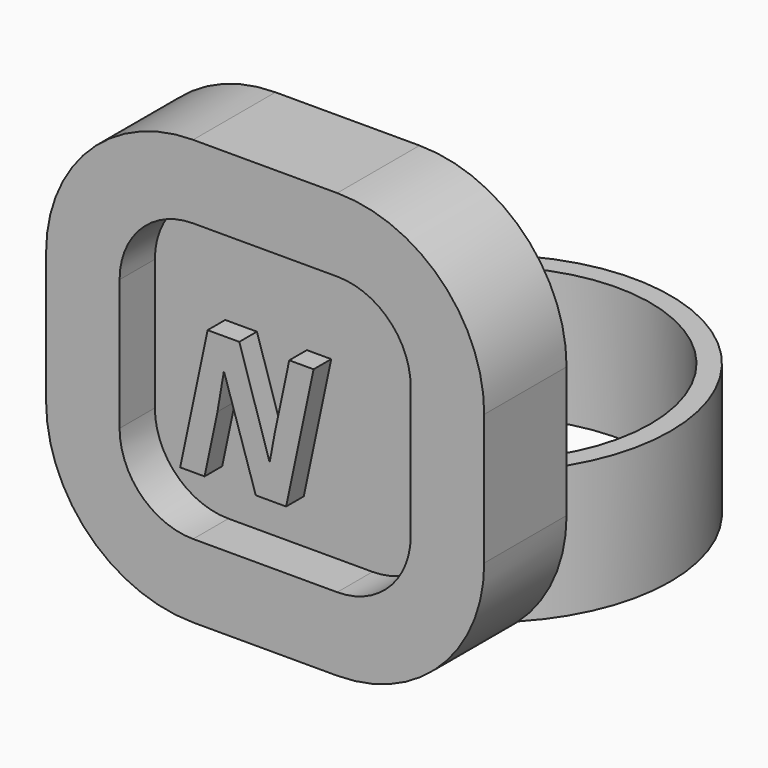
from build123d import *

# Parameters (mm, degrees)
F1_DEPTH     = 7
F2_DEPTH     = 4
F3_TEXT_SIZE = 12.3611111111
F4_DEPTH     = 1.5
F5_R         = 12.5
F5_R_2       = 11.15
F6_DEPTH     = 9


# Not quite as in the source:
# - a feature of the source that left no trace in its solid (it failed there, or was rolled back) is left out
# - Text() gives the source's letters only with a copy of the font that has no kerning and outlines rounded to 1/6400 em; it was checked with that copy


with BuildPart() as f1:
    # F0 (on Front) → F1 (new body)
    with BuildSketch(Plane.XZ):
        with BuildLine():
            Line((-90.7631201082, 7.9620657489), (-100.5631201082, 7.9620657489))
            ThreePointArc((-100.5631201082, 7.9620657489), (-107.6341876851, 5.0331336581), (-110.5631197759, -2.0379339188))
            Line((-110.5631197759, -2.0379339188), (-110.5631197759, -10.9379339188))
            ThreePointArc((-110.5631197759, -10.9379339188), (-107.6341876851, -18.0090014957), (-100.5631201082, -20.9379335865))
            Line((-100.5631201082, -20.9379335865), (-90.7631201082, -20.9379335865))
            ThreePointArc((-90.7631201082, -20.9379335865), (-83.6920525313, -18.0090014957), (-80.7631204405, -10.9379339188))
            Line((-80.7631204405, -10.9379339188), (-80.7631204405, -2.0379339188))
            ThreePointArc((-80.7631204405, -2.0379339188), (-83.6920525313, 5.0331336581), (-90.7631201082, 7.9620657489))
        make_face()
        with BuildLine():
            Line((-90.7631201082, -15.9379339188), (-100.5631201082, -15.9379339188))
            ThreePointArc((-100.5631201082, -15.9379339188), (-104.0986540141, -14.4734678248), (-105.5631201082, -10.9379339188))
            Line((-105.5631201082, -10.9379339188), (-105.5631201082, -2.0379339188))
            ThreePointArc((-105.5631201082, -2.0379339188), (-104.0986540141, 1.4975999871), (-100.5631201082, 2.9620660812))
            Line((-100.5631201082, 2.9620660812), (-90.7631201082, 2.9620660812))
            ThreePointArc((-90.7631201082, 2.9620660812), (-87.2275862022, 1.4975999871), (-85.7631201082, -2.0379339188))
            Line((-85.7631201082, -2.0379339188), (-85.7631201082, -10.9379339188))
            ThreePointArc((-85.7631201082, -10.9379339188), (-87.2275862022, -14.4734678248), (-90.7631201082, -15.9379339188))
        make_face(mode=Mode.SUBTRACT)
    extrude(amount=F1_DEPTH)

    # F0 (on Front) → F2 (join)
    with BuildSketch(Plane.XZ):
        with BuildLine():
            ThreePointArc((-105.5631201082, -10.9379339188), (-104.0986540141, -14.4734678248), (-100.5631201082, -15.9379339188))
            Line((-100.5631201082, -15.9379339188), (-90.7631201082, -15.9379339188))
            ThreePointArc((-90.7631201082, -15.9379339188), (-87.2275862022, -14.4734678248), (-85.7631201082, -10.9379339188))
            Line((-85.7631201082, -10.9379339188), (-85.7631201082, -2.0379339188))
            ThreePointArc((-85.7631201082, -2.0379339188), (-87.2275862022, 1.4975999871), (-90.7631201082, 2.9620660812))
            Line((-90.7631201082, 2.9620660812), (-100.5631201082, 2.9620660812))
            ThreePointArc((-100.5631201082, 2.9620660812), (-104.0986540141, 1.4975999871), (-105.5631201082, -2.0379339188))
            Line((-105.5631201082, -2.0379339188), (-105.5631201082, -10.9379339188))
        make_face()
    extrude(amount=F2_DEPTH)


with BuildPart() as f4:
    # F3 (on face) → F4 (new body)
    with BuildSketch(Plane.XZ.offset(7)):
        with Locations((-100.5631201082, -10.9379339188)):
            Text('N', F3_TEXT_SIZE, font='Open Sans', font_style=FontStyle.BOLDITALIC, text_align=(TextAlign.LEFT, TextAlign.BOTTOM))
    extrude(amount=F4_DEPTH)


with BuildPart() as f6:
    # F5 (on face) → F6 (new body)
    with BuildSketch(Plane(origin=(0, 0, -20.9379335865), x_dir=(1, 0, 0), z_dir=(0, 0, -1))):
        with Locations((-96.2080284953, -12.5091653317)):
            Circle(F5_R)
        with Locations((-96.2080284953, -12.5091653317)):
            Circle(F5_R_2, mode=Mode.SUBTRACT)
    extrude(amount=-F6_DEPTH)


solid = Compound([f1.part, f4.part, f6.part])
